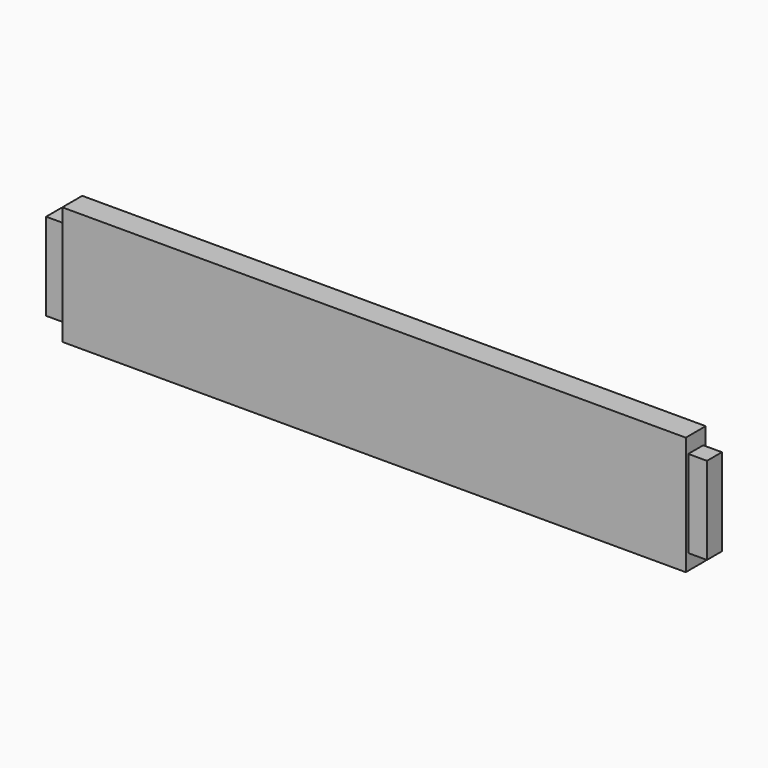
from build123d import *

# Parameters (mm, degrees)
F0_W     = 20
F0_H     = 95
F1_DEPTH = 250
F2_W     = 15
F2_H     = 70
F3_DEPTH = 15


# Not quite as in the source:
# - a pattern or mirror of a feature is missing from the dataset's text; its kind, count and spacing are read off the source's solid


with BuildPart() as f1:
    # F0 (on Right) → F1 (new body, symmetric)
    with BuildSketch(Plane.YZ):
        Rectangle(F0_W, F0_H)
    extrude(amount=F1_DEPTH, both=True)

    # F2 (on face) → F3 (join)
    with BuildSketch(Plane.YZ.offset(250)):
        Rectangle(F2_W, F2_H)
    f3 = extrude(amount=F3_DEPTH)

    # F3_copies: F3 across plane
    add(f3.mirror(Plane(origin=(0, 0, 0), x_dir=(0, 0, -1), z_dir=(-1, 0, 0))))


solid = f1.part
